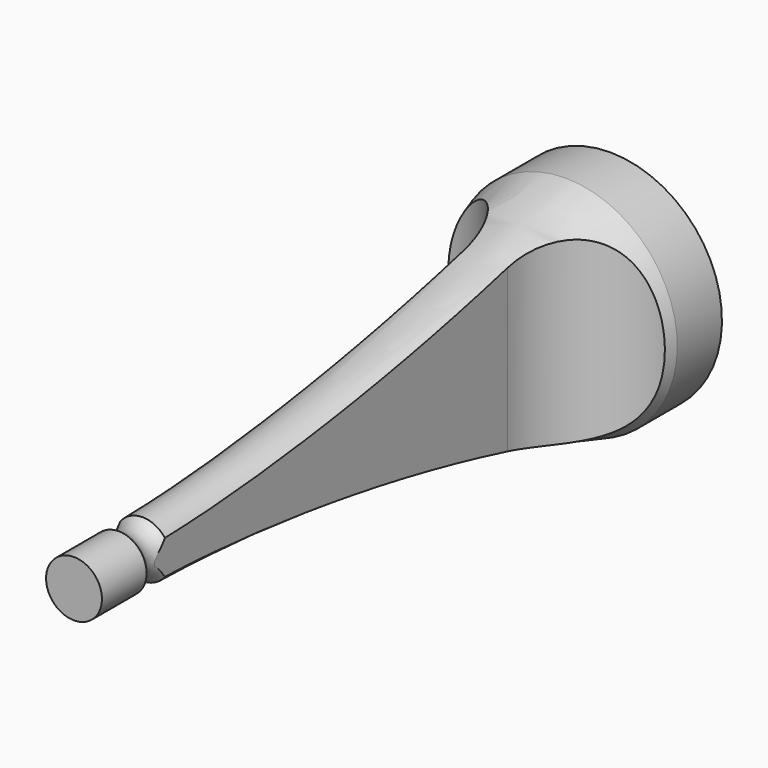
from build123d import *

# Parameters (mm, degrees)
F3_DEPTH      = 10.001
F3_DEPTH_BACK = 82


# Not quite as in the source:
# - an extrude ends at something that could not be found from the text; its depth is read off the source's solid


with BuildPart() as f1:
    # F0 (on Right) → F1 (revolve)
    with BuildSketch(Plane.YZ):
        with BuildLine():
            Line((-60, 0), (0, 0))
            Line((0, 0), (0, 10))
            Line((0, 10), (-5, 10))
            ThreePointArc((-5, 10), (-28.4012730043, 4.5885703785), (-52.3309178064, 2.5209029927))
            ThreePointArc((-52.3309178064, 2.5209029927), (-53.6614617682, 2.00006133), (-55, 2.5))
            Line((-55, 2.5), (-60, 2.5))
            Line((-60, 2.5), (-60, 0))
        make_face()
    revolve(axis=Axis((0, -19.4839663044, 0), (0, -1, 0)))

    # F2 (on Top) → F3 (cut, two sides)
    with BuildSketch(Plane.XY) as f3_sk:
        with BuildLine():
            Line((2, -14), (2, -53.5))
            Line((2, -53.5), (10, -53.5))
            Line((10, -53.5), (10, -6))
            ThreePointArc((10, -6), (4.3431457505, -8.3431457505), (2, -14))
        make_face()
        with BuildLine():
            Line((-10, -53.5), (-2, -53.5))
            Line((-2, -53.5), (-2, -14))
            ThreePointArc((-2, -14), (-4.3431457505, -8.3431457505), (-10, -6))
            Line((-10, -6), (-10, -53.5))
        make_face()
    extrude(amount=-F3_DEPTH, mode=Mode.SUBTRACT)
    extrude(f3_sk.sketch, amount=F3_DEPTH_BACK, mode=Mode.SUBTRACT)


solid = f1.part
